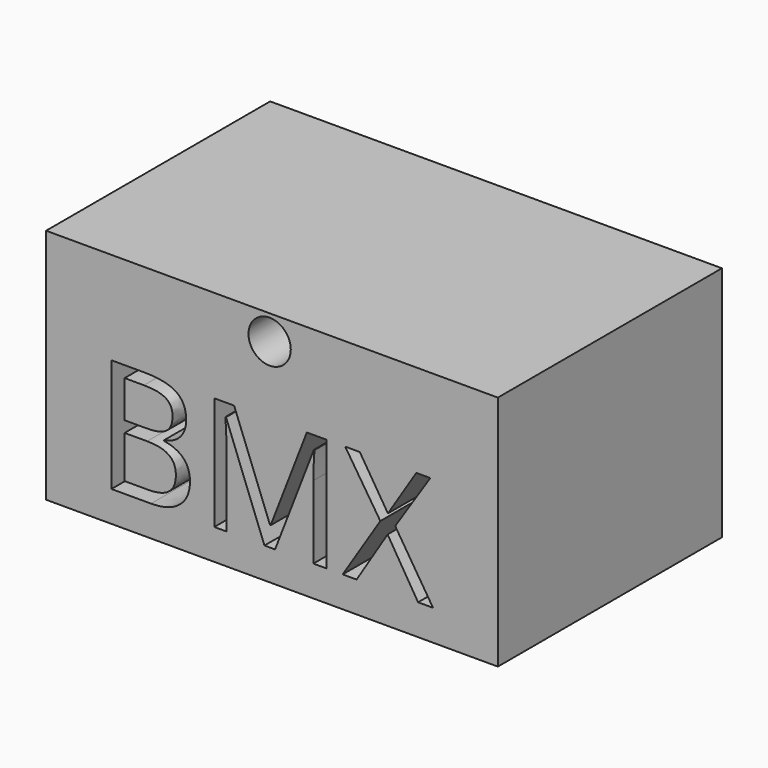
from build123d import *

# Parameters (mm, degrees)
F0_W         = 12.7
F0_H         = 6.6582536268
F3_DEPTH     = 7.874
F2_TEXT_SIZE = 4.4624321163
F4_DEPTH     = 25.4
F5_R         = 0.5945361401
F6_DEPTH     = 25.4


# Not quite as in the source:
# - Text() gives the source's letters only with a copy of the font that has no kerning and outlines rounded to 1/6400 em; it was checked with that copy


with BuildPart() as f3:
    # F0 (on Front) → F3 (new body)
    with BuildSketch(Plane.XZ):
        with Locations((-61.998270452, 60.7658904046)):
            Rectangle(F0_W, F0_H)
    extrude(amount=-F3_DEPTH)

    # F2 (on face) → F4 (cut)
    with BuildSketch(Plane.XZ):
        with Locations((-66.9488012791, 58.3004616201)):
            Text('BMX', F2_TEXT_SIZE, font='Open Sans', text_align=(TextAlign.LEFT, TextAlign.BOTTOM))
    extrude(amount=-F4_DEPTH, mode=Mode.SUBTRACT)

    # F5 (on face) → F6 (cut)
    with BuildSketch(Plane.XZ):
        with Locations((-62.0641261339, 63.3926987648)):
            Circle(F5_R)
    extrude(amount=-F6_DEPTH, mode=Mode.SUBTRACT)


solid = f3.part
